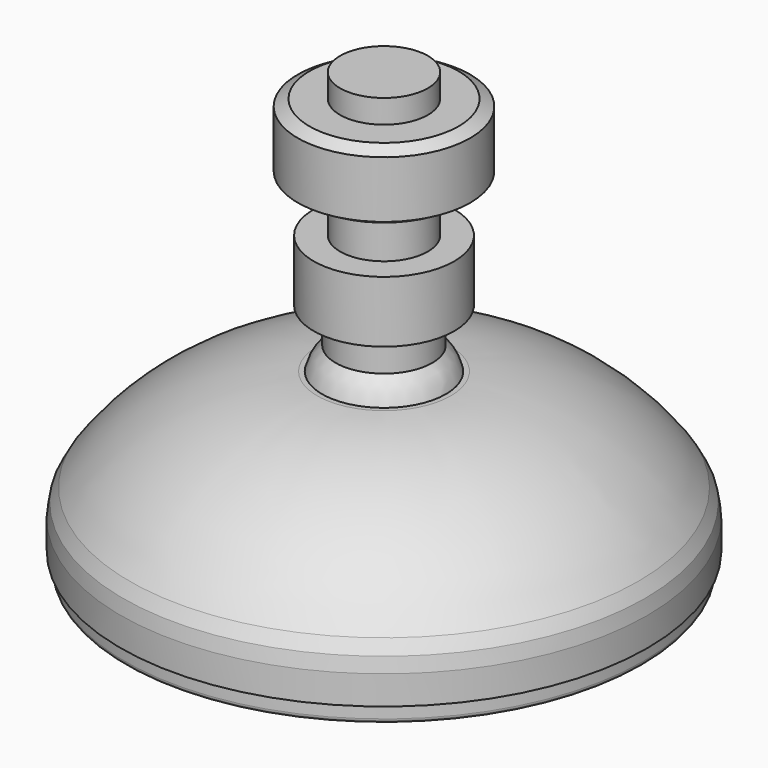
from build123d import *


# Not quite as in the source:
# - ends of sketch curves that miss each other by under 0.0002 mm in the source are joined


with BuildPart() as f1:
    # F0 (on Front) → F1 (revolve)
    with BuildSketch(Plane.XZ):
        with BuildLine():
            Line((-7.3999762, -4.999923), (-7.9499112, -4.999876))
            ThreePointArc((-7.9499112, -4.999876), (-8.5406711809, -3.5422157753), (-9.5911861302, -2.3716649112))
            Line((-9.5911861302, -2.3716649112), (-9.4998722, -2.374884))
            Line((-9.4998722, -2.374884), (-9.4998722, 1.625069))
            Line((-9.4998722, 1.625069), (-7.0000502, 1.625069))
            Line((-7.0000502, 1.625069), (-7.0000502, 8.625047))
            Line((-7.0000502, 8.625047), (-10.0000742, 8.625047))
            Line((-10.0000742, 8.625047), (-10.0000742, 14.321571))
            Line((-10.0000742, 14.321571), (-6.5000852, 14.321571))
            Line((-6.5000852, 14.321571), (-5.1849672, 15.080816))
            Line((-5.1849672, 15.080816), (-5.1849672, 21.562471))
            Line((-5.1849672, 21.562471), (-6.5000852, 22.321597))
            Line((-6.5000852, 22.321597), (-10.0000742, 22.321597))
            Line((-10.0000742, 22.321597), (-10.0000742, 25))
            Line((-10.0000742, 25), (-15.0000762, 25))
            Line((-15.0000762, 25), (-15.0000697718, 22.3215925))
            Line((-15.0000697718, 22.3215925), (-15.0000505717, 14.3215729999))
            Line((-15.0000505717, 14.3215729999), (-14.9999562, -25))
            Line((-14.9999562, -25), (4.9999238, -25))
            Line((4.9999238, -25), (14.0001218, -25))
            ThreePointArc((14.0001218, -25), (14.3536028976, -24.8535000977), (14.5000498, -24.499946))
            Line((14.5000498, -24.499946), (14.5000868, -22.999904))
            Line((14.5000868, -22.999904), (15.0000508, -22.999904))
            Line((15.0000508, -22.999904), (15.0000508, -19.719976))
            Line((15.0000508, -19.719976), (14.7301608, -18.099323))
            Line((14.7301608, -18.099323), (13.9495778, -16.653671))
            ThreePointArc((13.9495778, -16.653671), (4.6062496949, -8.3875220734), (-7.3999762, -4.999923))
        make_face()
    revolve(axis=Axis((-15.0000162, 0, 0), (2.4e-06, 0, -1)))


solid = f1.part
